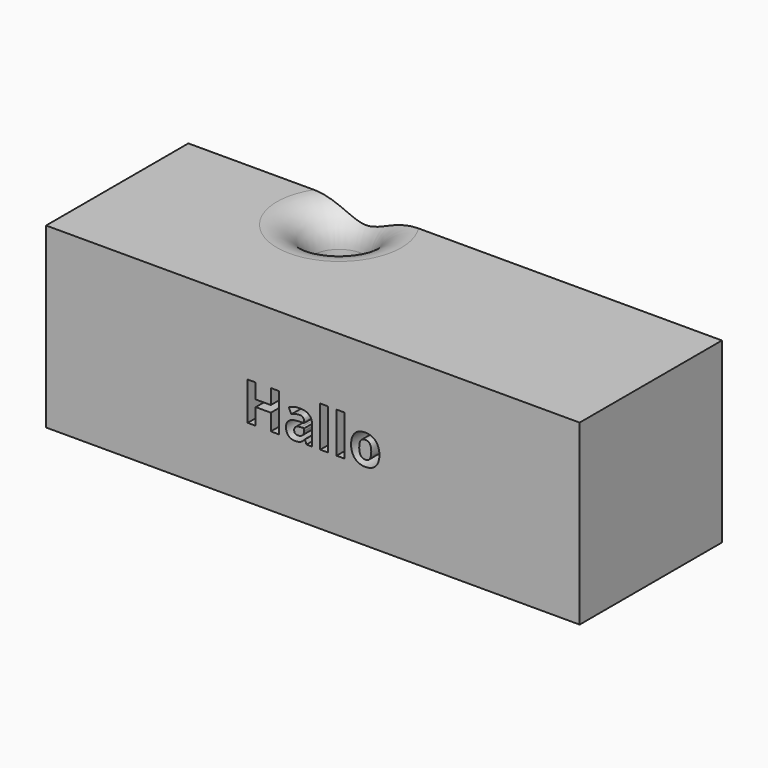
from build123d import *

# Parameters (mm, degrees)
F0_W           = 76.2
F0_H           = 25.4
F0_R           = 3.81
F1_DEPTH       = 25.4
F2_TEXT_SIZE   = 7.6376872128
F3_DEPTH       = 20
F5_D           = 4.4
F5_DEPTH       = 10.16
F5_CBORE_D     = 8.25
F5_CBORE_DEPTH = 4
F5_TIP         = 1.3218933619


# Not quite as in the source:
# - a fillet or chamfer that OpenCascade refuses, or shapes differently, is made with other operations: its cross-section is extruded or revolved along the edge and cut away or added
# - Text() gives the source's letters only with a copy of the font that has no kerning and outlines rounded to 1/6400 em; it was checked with that copy


with BuildPart() as f1:
    # F0 (on Top) → F1 (new body)
    with BuildSketch(Plane.XY):
        with Locations((-24.9147186286, -12.7)):
            Rectangle(F0_W, F0_H)
        with Locations((-37.6147186286, -4.8315519816)):
            Circle(F0_R, mode=Mode.SUBTRACT)
    extrude(amount=F1_DEPTH)

    # F2 (on face) → F3 (cut)
    with BuildSketch(Plane.XZ.offset(25.4)):
        with Locations((-34.9147186286, 9.9504326034)):
            Text('Hallo', F2_TEXT_SIZE, font='Open Sans', font_style=FontStyle.BOLD, text_align=(TextAlign.LEFT, TextAlign.BOTTOM))
    extrude(amount=-F3_DEPTH, mode=Mode.SUBTRACT)

    # F5
    with Locations(Plane(origin=(-63.0147186286, 0, 0), x_dir=(0, -1, 0), z_dir=(-1, 0, 0))):
        with Locations((8.7910248601, 16.2030365318), (18.9510248601, 6.0430365318), (8.7910248601, 6.0430365318), (18.9510248601, 16.2030365318)):
            CounterBoreHole(F5_D / 2, F5_CBORE_D / 2, F5_CBORE_DEPTH, depth=F5_DEPTH)
            with Locations((0, 0, -(F5_DEPTH + F5_TIP / 2))):  # 118° drill point
                Cone(0, F5_D / 2, F5_TIP, mode=Mode.SUBTRACT)

    # F6: fillet of radius 5.08 on 1 edges, made by hand

    # F6_s1 → F6_t2 (revolve, cut)
    with BuildSketch(Plane.XZ.offset(4.8315519816)):
        with BuildLine():
            ThreePointArc((-28.7247186286, 25.4), (-32.3168210771, 23.9121024484), (-33.8047186286, 20.32))
            Line((-33.8047186286, 20.32), (-33.8047186286, 25.4))
            Line((-33.8047186286, 25.4), (-28.7247186286, 25.4))
        make_face()
    revolve(axis=Axis((-37.6147186286, -4.8315519816, 25.4), (0, 0, 1)), mode=Mode.SUBTRACT)


solid = f1.part
